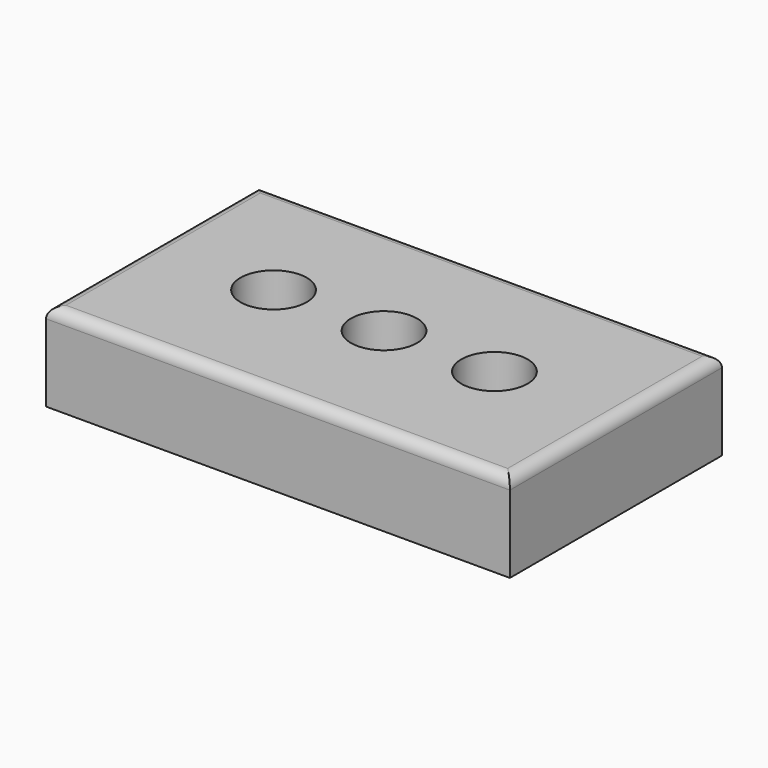
from build123d import *

# Parameters (mm, degrees)
F0_W     = 266.7
F0_H     = 152.4
F0_R     = 19.05
F1_DEPTH = 50.8
F2_DEPTH = 50.8
F3_R     = 6.35


with BuildPart() as f1:
    # F0 (on Top) → F1 (new body)
    with BuildSketch(Plane.XY):
        Rectangle(F0_W, F0_H)
        with Locations((-63.5, 0)):
            Circle(F0_R, mode=Mode.SUBTRACT)
        with BuildLine():
            ThreePointArc((-19.05, 0), (0, 19.05), (19.05, 0))
            ThreePointArc((19.05, 0), (0, -19.05), (-19.05, 0))
        make_face(mode=Mode.SUBTRACT)
        with BuildLine():
            ThreePointArc((82.55, 0), (63.5, -19.05), (44.45, 0))
            ThreePointArc((44.45, 0), (63.5, 19.05), (82.55, 0))
        make_face(mode=Mode.SUBTRACT)
    extrude(amount=-F1_DEPTH)

    # F0 (on Top) → F2 (cut)
    with BuildSketch(Plane.XY):
        with BuildLine():
            ThreePointArc((82.55, 0), (63.5, 19.05), (44.45, 0))
            ThreePointArc((44.45, 0), (63.5, -19.05), (82.55, 0))
        make_face()
        with Locations((-63.5, 0)):
            Circle(F0_R)
    extrude(amount=-F2_DEPTH, mode=Mode.SUBTRACT)

    # F3
    f3_edges = [f1.edges().sort_by_distance(p)[0] for p in [
        (0, 76.2, 0),
        (-133.35, 0, 0),
        (133.35, 0, 0),
        (0, -76.2, 0),
    ]]
    fillet(f3_edges, radius=F3_R)


solid = f1.part
